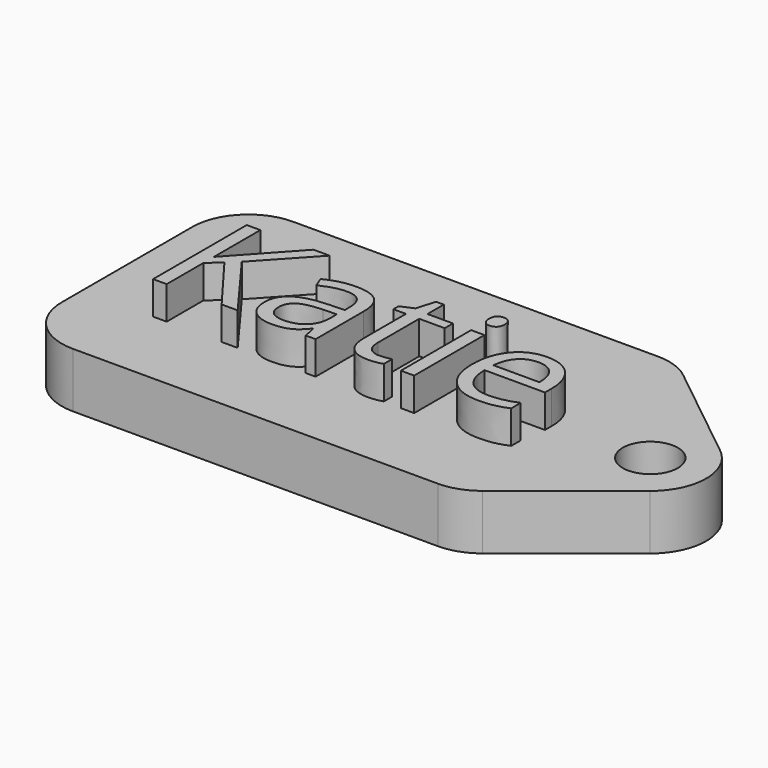
from build123d import *

# Parameters (mm, degrees)
F1_DEPTH     = 5
F2_R         = 5.08
F3_R         = 5.08
F5_D         = 5
F6_TEXT_SIZE = 14.8975791434
F7_DEPTH     = 3


# Not quite as in the source:
# - Text() gives the source's letters only with a copy of the font that has no kerning and outlines rounded to 1/6400 em; it was checked with that copy


with BuildPart() as f1:
    # F0 (on Top) → F1 (new body)
    with BuildSketch(Plane.XY):
        Polygon((-20, -12.5), (20, -12.5), (35.6578566134, 0), (20, 12.5), (-20, 12.5), align=None)
    extrude(amount=F1_DEPTH)

    # F2
    f2_edges = [f1.edges().sort_by_distance(p)[0] for p in [
        (35.657857, 0, 2.5),
    ]]
    fillet(f2_edges, radius=F2_R)

    # F3
    f3_edges = [f1.edges().sort_by_distance(p)[0] for p in [
        (20, -12.5, 2.5),
        (-20, -12.5, 2.5),
        (-20, 12.5, 2.5),
        (20, 12.5, 2.5),
    ]]
    fillet(f3_edges, radius=F3_R)

    # F5 (through all)
    with Locations(Plane.XY.offset(5)):
        with Locations((27.5154576744, 0)):
            Hole(F5_D / 2)

    # F6 (on face) → F7 (join)
    with BuildSketch(Plane.XY.offset(5)):
        with Locations((-15.027804419, -5.0891910523)):
            Text('Katie', F6_TEXT_SIZE, font='Open Sans', text_align=(TextAlign.LEFT, TextAlign.BOTTOM))
    extrude(amount=F7_DEPTH)


solid = f1.part
